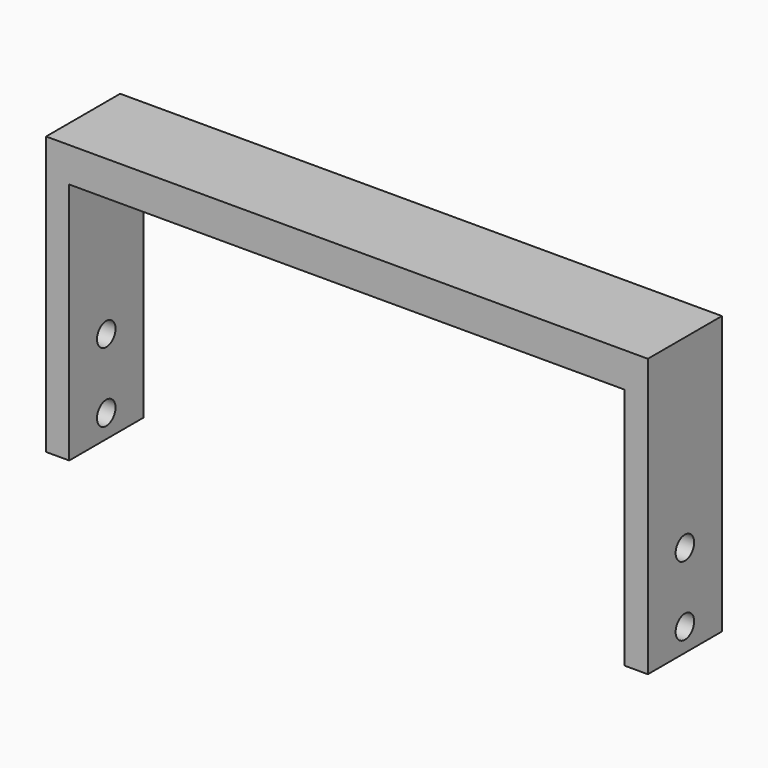
from build123d import *

# Parameters (mm, degrees)
F0_W     = 304.8
F0_H     = 50.8
F1_DEPTH = 19.05
F2_W     = 50.8
F2_H     = 152.4
F3_DEPTH = 12.7
F4_R     = 6.35
F5_DEPTH = 12.7


# Not quite as in the source:
# - a pattern or mirror of a feature is missing from the dataset's text; its kind, count and spacing are read off the source's solid


with BuildPart() as f1:
    # F0 (on Top) → F1 (new body)
    with BuildSketch(Plane.XY):
        Rectangle(F0_W, F0_H)
    extrude(amount=F1_DEPTH)

    # F2 (on face) → F3 (join)
    with BuildSketch(Plane.YZ.offset(152.4)):
        with Locations((0, -57.15)):
            Rectangle(F2_W, F2_H)
    f3 = extrude(amount=F3_DEPTH)

    # F3_copies: F3 across plane
    add(f3.mirror(Plane(origin=(0, 0, 0), x_dir=(0, 0, -1), z_dir=(-1, 0, 0))))

    # F4 (on face) → F5 (cut, through all)
    with BuildSketch(Plane.YZ.offset(165.1)):
        with Locations((0, -120.65)):
            Circle(F4_R)
        with Locations((0, -82.55)):
            Circle(F4_R)
    f5 = extrude(amount=-F5_DEPTH, mode=Mode.SUBTRACT)

    # F5_copies: F5 across plane
    add(f5.mirror(Plane(origin=(0, 0, 0), x_dir=(0, 0, -1), z_dir=(-1, 0, 0))), mode=Mode.SUBTRACT)


solid = f1.part
